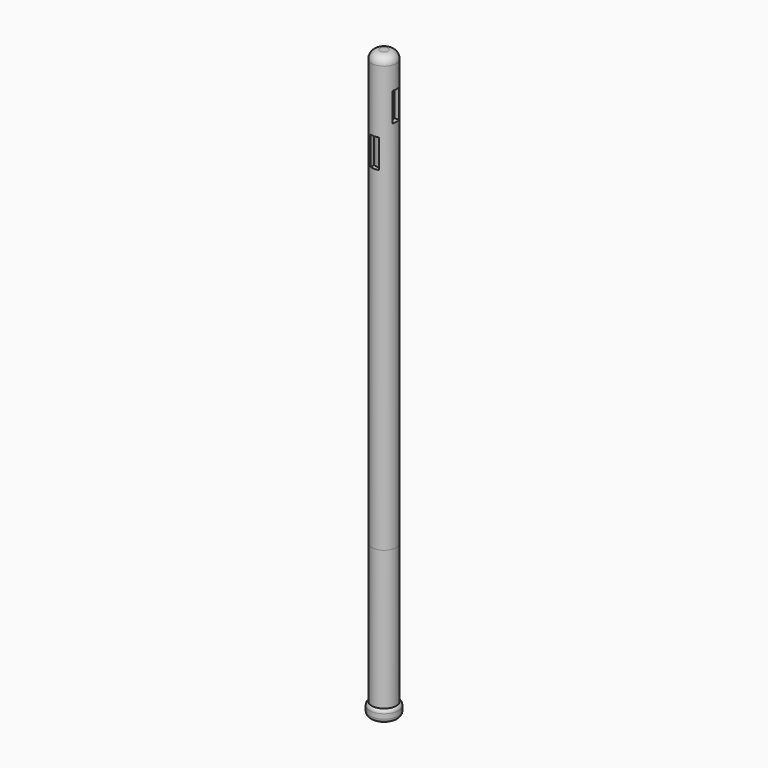
from build123d import *

# Parameters (mm, degrees)
F0_R      = 3
F0_R_2    = 2
F1_DEPTH  = 100
F2_R      = 3
F2_R_2    = 2
F3_DEPTH  = 6
F4_W      = 2
F4_H      = 7
F6_DEPTH  = 12.5
F5_W      = 2
F5_H      = 7
F7_DEPTH  = 12.5
F8_R      = 2
F9_DEPTH  = 34
F10_R     = 3.5
F10_R_2   = 3
F10_R_3   = 2
F11_DEPTH = 3


# Not quite as in the source:
# - a fillet or chamfer that OpenCascade refuses, or shapes differently, is made with other operations: its cross-section is extruded or revolved along the edge and cut away or added


with BuildPart() as f1:
    # F0 (on Top) → F1 (new body)
    with BuildSketch(Plane.XY):
        Circle(F0_R)
        Circle(F0_R_2, mode=Mode.SUBTRACT)
    extrude(amount=F1_DEPTH)

    # F2 (on face) → F3 (join)
    with BuildSketch(Plane.XY.offset(100)):
        Circle(F2_R)
        Circle(F2_R_2, mode=Mode.SUBTRACT)
        Circle(F2_R_2)
    extrude(amount=F3_DEPTH)

    # F4 (on Front) → F6 (cut, symmetric)
    with BuildSketch(Plane.XZ):
        with Locations((0, 85.1259604096)):
            Rectangle(F4_W, F4_H)
    extrude(amount=F6_DEPTH, both=True, mode=Mode.SUBTRACT)

    # F5 (on Right) → F7 (cut, symmetric)
    with BuildSketch(Plane.YZ):
        with Locations((0, 94.9563682079)):
            Rectangle(F5_W, F5_H)
    extrude(amount=F7_DEPTH, both=True, mode=Mode.SUBTRACT)

    # F8
    f8_edges = [f1.edges().sort_by_distance(p)[0] for p in [
        (-3, 0, 106),
    ]]
    fillet(f8_edges, radius=F8_R)

    # F9 (add): a face of the model
    f9_faces = [f1.faces().sort_by_distance(p)[0] for p in [
        (-2.9151471863, 0, 0),
    ]]
    extrude(f9_faces, amount=F9_DEPTH)

    # F10 (on face) → F11 (join)
    with BuildSketch(Plane(origin=(0, 0, -34), x_dir=(1, 0, 0), z_dir=(0, 0, -1))):
        Circle(F10_R)
        Circle(F10_R_2, mode=Mode.SUBTRACT)
        Circle(F10_R_2)
        Circle(F10_R_3, mode=Mode.SUBTRACT)
    extrude(amount=F11_DEPTH)

    # F12: fillet of radius 1 on 2 edges, made by hand

    # F12_s1 → F12_t2 (revolve, cut)
    with BuildSketch(Plane.XZ):
        with BuildLine():
            ThreePointArc((3, -34), (3.3660254038, -34.3660254038), (3.5, -34.8660254038))
            Line((3.5, -34.8660254038), (3.5, -34))
            Line((3.5, -34), (3, -34))
        make_face()
    revolve(axis=Axis((0, 0, -34), (0, 0, -1)), mode=Mode.SUBTRACT)

    # F12_s3 → F12_t4 (revolve, cut)
    with BuildSketch(Plane.XZ):
        with BuildLine():
            ThreePointArc((3.5, -36), (3.2071067812, -36.7071067812), (2.5, -37))
            Line((2.5, -37), (3.5, -37))
            Line((3.5, -37), (3.5, -36))
        make_face()
    revolve(axis=Axis((0, 0, -37), (0, 0, -1)), mode=Mode.SUBTRACT)


solid = f1.part
